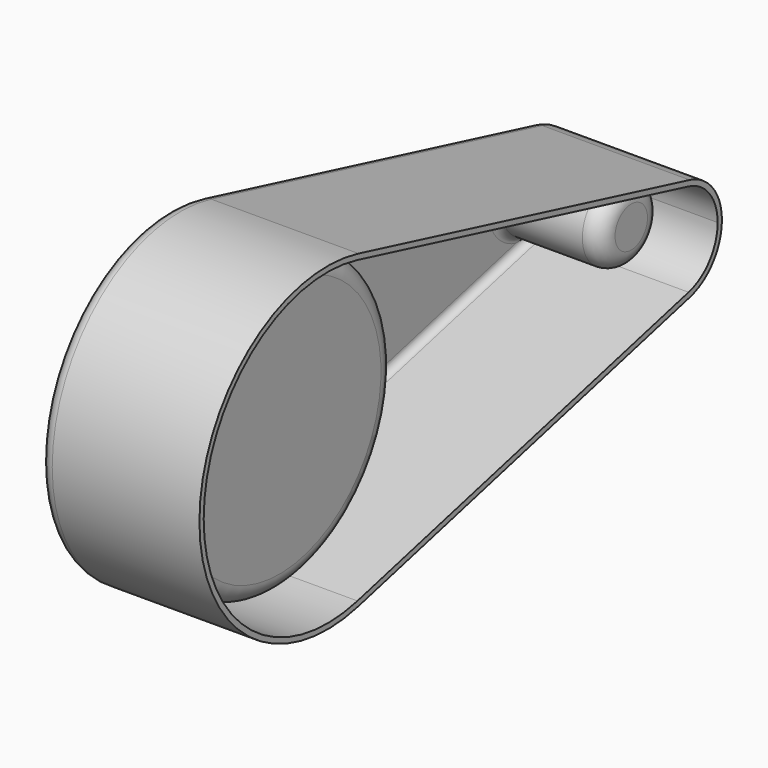
from build123d import *

# Parameters (mm, degrees)
F1_DEPTH     = 75
F2_R         = 65.5
F2_R_2       = 15.5
F3_DEPTH     = 50
F4_T5_DEPTH  = 200
F4_T7_DEPTH  = 200
F4_T10_ANGLE = 151.9275130641
F4_T12_ANGLE = 208.0724869359
F5_T         = -2.5


# Not quite as in the source:
# - a fillet or chamfer that OpenCascade refuses, or shapes differently, is made with other operations: its cross-section is extruded or revolved along the edge and cut away or added


with BuildPart() as f1:
    # F0 (on Right) → F1 (new body)
    with BuildSketch(Plane.YZ):
        with BuildLine():
            ThreePointArc((18.1901718777, 72.7606875109), (59.1154078512, 46.1559157052), (75, 0))
            ThreePointArc((75, 0), (59.1154078512, -46.1559157052), (18.1901718777, -72.7606875109))
            Line((18.1901718777, -72.7606875109), (212.2186719068, -24.2535625036))
            ThreePointArc((212.2186719068, -24.2535625036), (181.1552812809, 0), (212.2186719068, 24.2535625036))
            Line((212.2186719068, 24.2535625036), (18.1901718777, 72.7606875109))
        make_face()
        with BuildLine():
            ThreePointArc((18.1901718777, -72.7606875109), (59.1154078512, -46.1559157052), (75, 0))
            ThreePointArc((75, 0), (59.1154078512, 46.1559157052), (18.1901718777, 72.7606875109))
            ThreePointArc((18.1901718777, 72.7606875109), (-75, 0), (18.1901718777, -72.7606875109))
        make_face()
        with BuildLine():
            ThreePointArc((231.1552812809, 0), (225.8604172313, 15.3853052351), (212.2186719068, 24.2535625036))
            ThreePointArc((212.2186719068, 24.2535625036), (181.1552812809, 0), (212.2186719068, -24.2535625036))
            ThreePointArc((212.2186719068, -24.2535625036), (225.8604172313, -15.3853052351), (231.1552812809, 0))
        make_face()
    extrude(amount=F1_DEPTH)

    # F2 (on face) → F3 (cut)
    with BuildSketch(Plane(origin=(0, 0, 0), x_dir=(0, -1, 0), z_dir=(-1, 0, 0))):
        Circle(F2_R)
        with Locations((-206.1552812809, 0)):
            Circle(F2_R_2)
    extrude(amount=-F3_DEPTH, mode=Mode.SUBTRACT)

    # F4: fillet of radius 6 on 8 edges, made by hand

    # F4_s1 → F4_t2 (revolve)
    with BuildSketch(Plane.XY):
        with BuildLine():
            ThreePointArc((44, -65.5), (48.2426406871, -63.7426406871), (50, -59.5))
            Line((50, -59.5), (50.12, -59.5))
            Line((50.12, -59.5), (50.12, -65.62))
            Line((50.12, -65.62), (44, -65.62))
            Line((44, -65.62), (44, -65.5))
        make_face()
    revolve(axis=Axis((50, 0, 0), (-1, 0, 0)))

    # F4_s3 → F4_t4 (revolve)
    with BuildSketch(Plane.XY):
        with BuildLine():
            ThreePointArc((44, 190.6552812809), (48.2426406871, 192.4126405938), (50, 196.6552812809))
            Line((50, 196.6552812809), (50.12, 196.6552812809))
            Line((50.12, 196.6552812809), (50.12, 190.5352812809))
            Line((50.12, 190.5352812809), (44, 190.5352812809))
            Line((44, 190.5352812809), (44, 190.6552812809))
        make_face()
    revolve(axis=Axis((50, 206.1552812809, 0), (-1, 0, 0)))

    # F4_s6 → F4_t5 (cut)
    with BuildSketch(Plane(origin=(0, 194.0285000291, -48.5071250073), x_dir=(1, 0, 0), z_dir=(0, -0.9701425001, 0.242535625))):
        with BuildLine():
            ThreePointArc((6, 75), (1.7573593129, 73.2426406871), (0, 69))
            Line((0, 69), (-0.12, 69))
            Line((-0.12, 69), (-0.12, 75.12))
            Line((-0.12, 75.12), (6, 75.12))
            Line((6, 75.12), (6, 75))
        make_face()
    extrude(amount=F4_T5_DEPTH, mode=Mode.SUBTRACT)

    # F4_s8 → F4_t7 (cut)
    with BuildSketch(Plane(origin=(0, 0, 0), x_dir=(1, 0, 0), z_dir=(0, 0.9701425001, 0.242535625))):
        with BuildLine():
            ThreePointArc((0, 69), (1.7573593129, 73.2426406871), (6, 75))
            Line((6, 75), (6, 75.12))
            Line((6, 75.12), (-0.12, 75.12))
            Line((-0.12, 75.12), (-0.12, 69))
            Line((-0.12, 69), (0, 69))
        make_face()
    extrude(amount=F4_T7_DEPTH, mode=Mode.SUBTRACT)

    # F4_s9 → F4_t10 (revolve, cut)
    with BuildSketch(Plane(origin=(0, 194.0285000291, 48.5071250073), x_dir=(1, 0, 0), z_dir=(0, -0.9701425001, -0.242535625))):
        with BuildLine():
            ThreePointArc((6, -75), (1.7573593129, -73.2426406871), (0, -69))
            Line((0, -69), (-0.12, -69))
            Line((-0.12, -69), (-0.12, -75.12))
            Line((-0.12, -75.12), (6, -75.12))
            Line((6, -75.12), (6, -75))
        make_face()
    revolve(axis=Axis((0, 206.1552812809, 0), (1, 0, 0)), revolution_arc=F4_T10_ANGLE, mode=Mode.SUBTRACT)

    # F4_s11 → F4_t12 (revolve, cut)
    with BuildSketch(Plane(origin=(0, 0, 0), x_dir=(1, 0, 0), z_dir=(0, 0.9701425001, -0.242535625))):
        with BuildLine():
            ThreePointArc((6, -75), (1.7573593129, -73.2426406871), (0, -69))
            Line((0, -69), (-0.12, -69))
            Line((-0.12, -69), (-0.12, -75.12))
            Line((-0.12, -75.12), (6, -75.12))
            Line((6, -75.12), (6, -75))
        make_face()
    revolve(axis=Axis((0, 0, 0), (1, 0, 0)), revolution_arc=F4_T12_ANGLE, mode=Mode.SUBTRACT)

    # F4_s13 → F4_t14 (revolve, cut)
    with BuildSketch(Plane.XY):
        with BuildLine():
            ThreePointArc((0, -71.5), (1.7573593129, -67.2573593129), (6, -65.5))
            Line((6, -65.5), (6, -65.38))
            Line((6, -65.38), (-0.12, -65.38))
            Line((-0.12, -65.38), (-0.12, -71.5))
            Line((-0.12, -71.5), (0, -71.5))
        make_face()
    revolve(axis=Axis((0, 0, 0), (-1, 0, 0)), mode=Mode.SUBTRACT)

    # F4_s15 → F4_t16 (revolve, cut)
    with BuildSketch(Plane.XY):
        with BuildLine():
            ThreePointArc((0, 184.6552812809), (1.7573593129, 188.897921968), (6, 190.6552812809))
            Line((6, 190.6552812809), (6, 190.7752812809))
            Line((6, 190.7752812809), (-0.12, 190.7752812809))
            Line((-0.12, 190.7752812809), (-0.12, 184.6552812809))
            Line((-0.12, 184.6552812809), (0, 184.6552812809))
        make_face()
    revolve(axis=Axis((0, 206.1552812809, 0), (-1, 0, 0)), mode=Mode.SUBTRACT)

    # F5
    f5_openings = [f1.faces().sort_by_distance(p)[0] for p in [
        (75, 56.613425, 0),
    ]]
    offset(amount=F5_T, openings=f5_openings)


solid = f1.part
